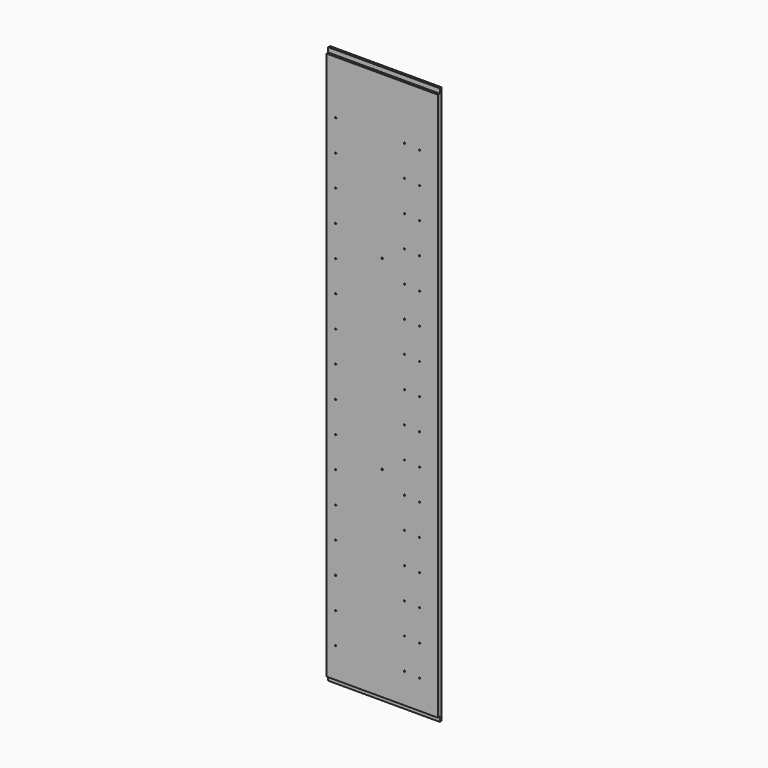
from build123d import *

# Parameters (mm, degrees)
F0_W           = 360
F0_H           = 1750
F1_DEPTH       = 15
F3_D           = 4
F3_DEPTH       = 5
F3_TIP         = 1.2017212381
F5_D           = 5.2
F5_DEPTH       = 15
F5_CBORE_D     = 15.5
F5_CBORE_DEPTH = 3
F5_TIP         = 1.5622376095
F7_W           = 7.5
F7_H           = 15
F8_DEPTH       = 360


# Not quite as in the source:
# - a pattern or mirror of a feature is missing from the dataset's text; its kind, count and spacing are read off the source's solid
# - a feature names something its author has since deleted; it is built from what else it names


with BuildPart() as f1:
    # F0 (on Front) → F1 (new body)
    with BuildSketch(Plane.XZ):
        with Locations((180, 875)):
            Rectangle(F0_W, F0_H)
    extrude(amount=F1_DEPTH)

    # F1_copies: F1 across plane


with BuildPart() as f1_1:
    add(f1.part)
    add(f1.part.mirror(Plane.XY.offset(900)))

    # F3
    with Locations(Plane.XZ.offset(15)):
        with Locations((252, 1612), (301, 408), (301, 508), (252, 412), (301, 1108), (252, 912), (301, 1408), (30, 412), (252, 612), (252, 1212), (30, 1012), (252, 1512), (30, 312), (252, 312), (301, 308), (30, 812), (30, 1312), (301, 1608), (252, 1112), (301, 1008), (30, 1612), (30, 712), (301, 908), (301, 108), (30, 512), (30, 1112), (252, 712), (30, 1212), (30, 212), (301, 1308), (252, 1412), (252, 1312), (301, 608), (30, 1512), (301, 808), (30, 112), (301, 708), (30, 612), (252, 512), (252, 1012), (252, 112), (301, 1208), (30, 1412), (30, 912), (301, 208), (252, 812), (301, 1508), (252, 212)):
            Hole(F3_D / 2, depth=F3_DEPTH)
            with Locations((0, 0, -(F3_DEPTH + F3_TIP / 2))):  # 118° drill point
                Cone(0, F3_D / 2, F3_TIP, mode=Mode.SUBTRACT)

    # F5
    with Locations(Plane(origin=(0, 0, 0), x_dir=(-1, 0, 0), z_dir=(0, 1, 0))):
        with Locations((-180, 1262), (-180, 662)):
            CounterBoreHole(F5_D / 2, F5_CBORE_D / 2, F5_CBORE_DEPTH, depth=F5_DEPTH)
            with Locations((0, 0, -(F5_DEPTH + F5_TIP / 2))):  # 118° drill point
                Cone(0, F5_D / 2, F5_TIP, mode=Mode.SUBTRACT)

    # F7 (on face) → F8 (cut, through all)
    with BuildSketch(Plane(origin=(0, 0, 0), x_dir=(0, -1, 0), z_dir=(-1, 0, 0))):
        with Locations((11.25, 7.5)):
            Rectangle(F7_W, F7_H)
    f8 = extrude(amount=-F8_DEPTH, mode=Mode.SUBTRACT)

    # F8_copies: F8 across plane
    add(f8.mirror(Plane.XY.offset(900)), mode=Mode.SUBTRACT)


solid = f1_1.part
